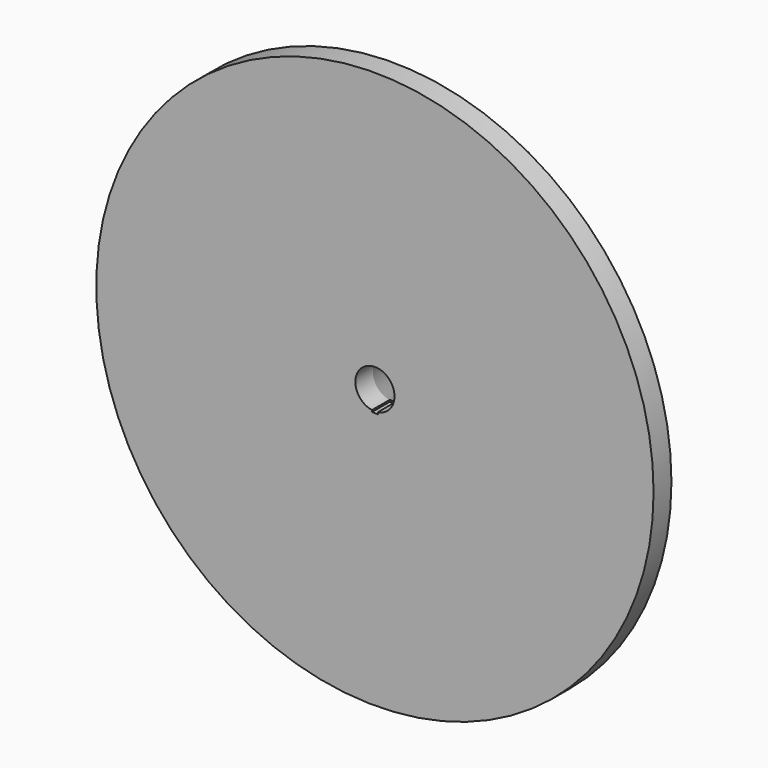
from build123d import *

# Parameters (mm, degrees)
F0_R     = 791.9998307979
F1_DEPTH = 63.5
F2_DEPTH = 127
F3_COUNT = 24
F3_ANGLE = 345


with BuildPart() as f1:
    # F0 (on Front) → F1 (new body)
    with BuildSketch(Plane.XZ):
        with Locations((-50.766086911, 60.2973892685)):
            Circle(F0_R)
        with BuildLine():
            ThreePointArc((-32.1512974758, 525.9283263062), (-31.2153070038, -405.2951868292), (-108.3512974758, 522.7285986786))
            add(Edge.make_bspline(
                [(-108.3512974758, 522.7285986786), (-97.9020277807, 568.3872993355), (-76.9030805915, 658.9701220312), (-47.0825344704, 570.6089033598), (-32.1512974758, 525.9283263062)],
                knots=[0, 0, 0, 0, 0.4992953447, 1, 1, 1, 1], degree=3))
        make_face(mode=Mode.SUBTRACT)
        with BuildLine():
            add(Edge.make_bspline(
                [(-108.3512974758, 522.7285986786), (-97.9020277807, 568.3872993355), (-76.9030805915, 658.9701220312), (-47.0825344704, 570.6089033598), (-32.1512974758, 525.9283263062)],
                knots=[0, 0, 0, 0, 0.4992953447, 1, 1, 1, 1], degree=3))
            ThreePointArc((-108.3512974758, 522.7285986786), (-31.2153070038, -405.2951868292), (-32.1512974758, 525.9283263062))
        make_face()
        with BuildLine():
            ThreePointArc((-59.021086911, 5.3089210428), (-50.766086911, 115.9020353227), (-42.511086911, 5.3089210428))
            Line((-42.511086911, 5.3089210428), (-42.511086911, 0))
            Line((-42.511086911, 0), (-59.021086911, 0.1983025765))
            Line((-59.021086911, 0.1983025765), (-59.021086911, 5.3089210428))
        make_face(mode=Mode.SUBTRACT)
    extrude(amount=F1_DEPTH)


with BuildPart() as f2:
    # F0 (on Front) → F2 (new body)
    with BuildSketch(Plane.XZ):
        with BuildLine():
            add(Edge.make_bspline(
                [(-108.3512974758, 522.7285986786), (-97.9020277807, 568.3872993355), (-76.9030805915, 658.9701220312), (-47.0825344704, 570.6089033598), (-32.1512974758, 525.9283263062)],
                knots=[0, 0, 0, 0, 0.4992953447, 1, 1, 1, 1], degree=3))
            ThreePointArc((-108.3512974758, 522.7285986786), (-31.2153070038, -405.2951868292), (-32.1512974758, 525.9283263062))
        make_face()
        with BuildLine():
            ThreePointArc((-59.021086911, 5.3089210428), (-50.766086911, 115.9020353227), (-42.511086911, 5.3089210428))
            Line((-42.511086911, 5.3089210428), (-42.511086911, 0))
            Line((-42.511086911, 0), (-59.021086911, 0.1983025765))
            Line((-59.021086911, 0.1983025765), (-59.021086911, 5.3089210428))
        make_face(mode=Mode.SUBTRACT)
    extrude(amount=-F2_DEPTH)


with BuildPart() as f3_1:
    # F3: instance of F2
    add(f2.part.rotate(Axis((-50.766086911, 0, 60.2973892685), (0, -1, 0)), 1 * F3_ANGLE / (F3_COUNT - 1)))


with BuildPart() as f3_2:
    # F3: instance of F2
    add(f2.part.rotate(Axis((-50.766086911, 0, 60.2973892685), (0, -1, 0)), 2 * F3_ANGLE / (F3_COUNT - 1)))


with BuildPart() as f3_3:
    # F3: instance of F2
    add(f2.part.rotate(Axis((-50.766086911, 0, 60.2973892685), (0, -1, 0)), 3 * F3_ANGLE / (F3_COUNT - 1)))


with BuildPart() as f3_4:
    # F3: instance of F2
    add(f2.part.rotate(Axis((-50.766086911, 0, 60.2973892685), (0, -1, 0)), 4 * F3_ANGLE / (F3_COUNT - 1)))


with BuildPart() as f3_5:
    # F3: instance of F2
    add(f2.part.rotate(Axis((-50.766086911, 0, 60.2973892685), (0, -1, 0)), 5 * F3_ANGLE / (F3_COUNT - 1)))


with BuildPart() as f3_6:
    # F3: instance of F2
    add(f2.part.rotate(Axis((-50.766086911, 0, 60.2973892685), (0, -1, 0)), 6 * F3_ANGLE / (F3_COUNT - 1)))


with BuildPart() as f3_7:
    # F3: instance of F2
    add(f2.part.rotate(Axis((-50.766086911, 0, 60.2973892685), (0, -1, 0)), 7 * F3_ANGLE / (F3_COUNT - 1)))


with BuildPart() as f3_8:
    # F3: instance of F2
    add(f2.part.rotate(Axis((-50.766086911, 0, 60.2973892685), (0, -1, 0)), 8 * F3_ANGLE / (F3_COUNT - 1)))


with BuildPart() as f3_9:
    # F3: instance of F2
    add(f2.part.rotate(Axis((-50.766086911, 0, 60.2973892685), (0, -1, 0)), 9 * F3_ANGLE / (F3_COUNT - 1)))


with BuildPart() as f3_10:
    # F3: instance of F2
    add(f2.part.rotate(Axis((-50.766086911, 0, 60.2973892685), (0, -1, 0)), 10 * F3_ANGLE / (F3_COUNT - 1)))


with BuildPart() as f3_11:
    # F3: instance of F2
    add(f2.part.rotate(Axis((-50.766086911, 0, 60.2973892685), (0, -1, 0)), 11 * F3_ANGLE / (F3_COUNT - 1)))


with BuildPart() as f3_12:
    # F3: instance of F2
    add(f2.part.rotate(Axis((-50.766086911, 0, 60.2973892685), (0, -1, 0)), 12 * F3_ANGLE / (F3_COUNT - 1)))


with BuildPart() as f3_13:
    # F3: instance of F2
    add(f2.part.rotate(Axis((-50.766086911, 0, 60.2973892685), (0, -1, 0)), 13 * F3_ANGLE / (F3_COUNT - 1)))


with BuildPart() as f3_14:
    # F3: instance of F2
    add(f2.part.rotate(Axis((-50.766086911, 0, 60.2973892685), (0, -1, 0)), 14 * F3_ANGLE / (F3_COUNT - 1)))


with BuildPart() as f3_15:
    # F3: instance of F2
    add(f2.part.rotate(Axis((-50.766086911, 0, 60.2973892685), (0, -1, 0)), 15 * F3_ANGLE / (F3_COUNT - 1)))


with BuildPart() as f3_16:
    # F3: instance of F2
    add(f2.part.rotate(Axis((-50.766086911, 0, 60.2973892685), (0, -1, 0)), 16 * F3_ANGLE / (F3_COUNT - 1)))


with BuildPart() as f3_17:
    # F3: instance of F2
    add(f2.part.rotate(Axis((-50.766086911, 0, 60.2973892685), (0, -1, 0)), 17 * F3_ANGLE / (F3_COUNT - 1)))


with BuildPart() as f3_18:
    # F3: instance of F2
    add(f2.part.rotate(Axis((-50.766086911, 0, 60.2973892685), (0, -1, 0)), 18 * F3_ANGLE / (F3_COUNT - 1)))


with BuildPart() as f3_19:
    # F3: instance of F2
    add(f2.part.rotate(Axis((-50.766086911, 0, 60.2973892685), (0, -1, 0)), 19 * F3_ANGLE / (F3_COUNT - 1)))


with BuildPart() as f3_20:
    # F3: instance of F2
    add(f2.part.rotate(Axis((-50.766086911, 0, 60.2973892685), (0, -1, 0)), 20 * F3_ANGLE / (F3_COUNT - 1)))


with BuildPart() as f3_21:
    # F3: instance of F2
    add(f2.part.rotate(Axis((-50.766086911, 0, 60.2973892685), (0, -1, 0)), 21 * F3_ANGLE / (F3_COUNT - 1)))


with BuildPart() as f3_22:
    # F3: instance of F2
    add(f2.part.rotate(Axis((-50.766086911, 0, 60.2973892685), (0, -1, 0)), 22 * F3_ANGLE / (F3_COUNT - 1)))


with BuildPart() as f3_23:
    # F3: instance of F2
    add(f2.part.rotate(Axis((-50.766086911, 0, 60.2973892685), (0, -1, 0)), 23 * F3_ANGLE / (F3_COUNT - 1)))


solid = Compound([f1.part, f2.part, f3_1.part, f3_2.part, f3_3.part, f3_4.part, f3_5.part, f3_6.part, f3_7.part, f3_8.part, f3_9.part, f3_10.part, f3_11.part, f3_12.part, f3_13.part, f3_14.part, f3_15.part, f3_16.part, f3_17.part, f3_18.part, f3_19.part, f3_20.part, f3_21.part, f3_22.part, f3_23.part])
